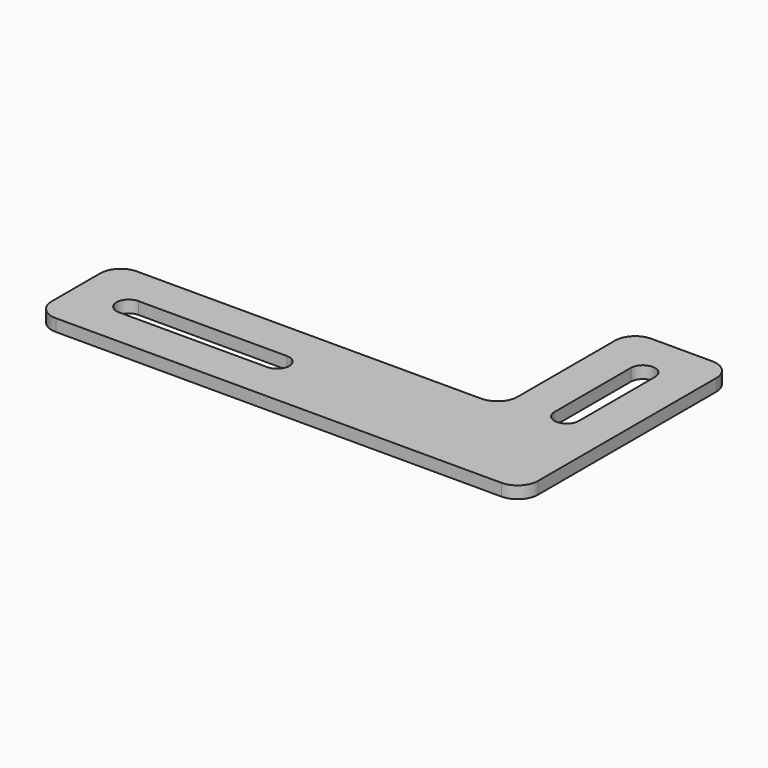
from build123d import *

# Parameters (mm, degrees)
F0_W     = 25
F0_H     = 40
F1_DEPTH = 3
F2_R     = 5


with BuildPart() as f1:
    # F0 (on Top) → F1 (new body)
    with BuildSketch(Plane.XY):
        Polygon((56.1464983402, 0), (-38.8535016598, 0), (-38.8535016598, -25), (81.1464983402, -25), (81.1464983402, 0), align=None)
        with BuildLine():
            ThreePointArc((-25.8535016598, -15.5), (-28.8535016598, -12.5), (-25.8535016598, -9.5))
            Line((-25.8535016598, -9.5), (10.752664879, -9.5))
            ThreePointArc((10.752664879, -9.5), (12.8739852225, -10.3786796564), (13.752664879, -12.5))
            ThreePointArc((13.752664879, -12.5), (12.8739852225, -14.6213203436), (10.752664879, -15.5))
            Line((10.752664879, -15.5), (-25.8535016598, -15.5))
        make_face(mode=Mode.SUBTRACT)
        with Locations((68.6464983402, 20)):
            Rectangle(F0_W, F0_H)
        with BuildLine():
            ThreePointArc((65.6464983402, 28), (68.6464983402, 31), (71.6464983402, 28))
            Line((71.6464983402, 28), (71.6464983402, 4.4783727005))
            ThreePointArc((71.6464983402, 4.4783727005), (68.6464983402, 1.4783727005), (65.6464983402, 4.4783727005))
            Line((65.6464983402, 4.4783727005), (65.6464983402, 28))
        make_face(mode=Mode.SUBTRACT)
    extrude(amount=F1_DEPTH)

    # F2
    f2_edges = [f1.edges().sort_by_distance(p)[0] for p in [
        (-38.853502, -25, 1.5),
        (81.146498, -25, 1.5),
        (-38.853502, 0, 1.5),
        (81.146498, 40, 1.5),
        (56.146498, 40, 1.5),
        (56.146498, 0, 1.5),
    ]]
    fillet(f2_edges, radius=F2_R)


solid = f1.part
